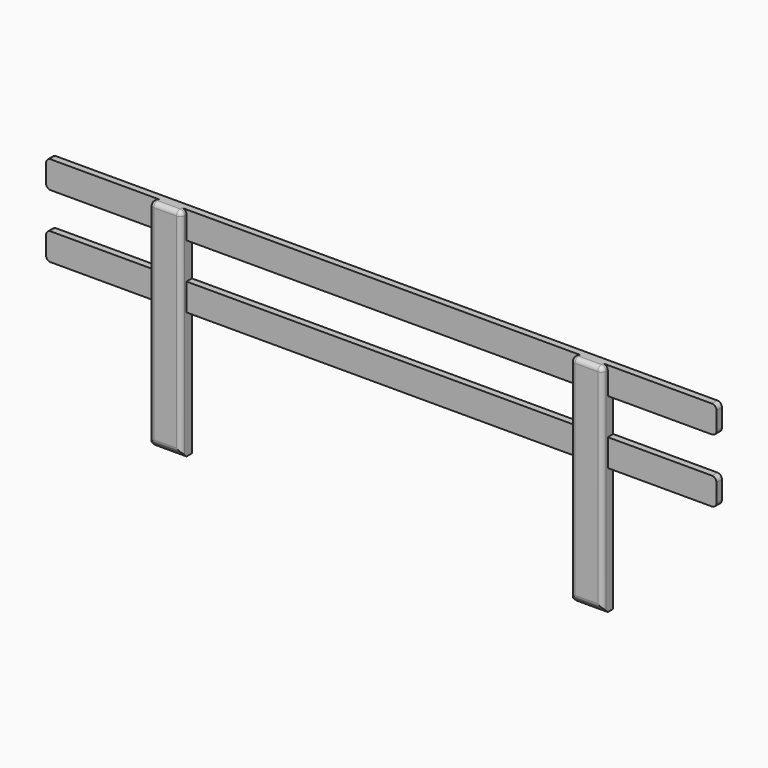
from build123d import *

# Parameters (mm, degrees)
F0_W     = 19.05
F0_H     = 76.2
F1_DEPTH = 939.8
F2_W     = 88.9
F2_H     = 38.1
F3_DEPTH = 609.6
F4_SIZE  = 19.05
F5_W     = 19.05
F5_H     = 76.2
F6_DEPTH = 939.8
F7_R     = 12.7


with BuildPart() as f1:
    # F0 (on Right) → F1 (new body, symmetric)
    with BuildSketch(Plane.YZ):
        with Locations((-9.525, 571.5)):
            Rectangle(F0_W, F0_H)
    extrude(amount=F1_DEPTH, both=True)

    # F2 (on face) → F3 (join, through all)
    with BuildSketch(Plane.XY.offset(609.6)):
        with Locations((590.55, -19.05)):
            Rectangle(F2_W, F2_H)
        with Locations((-590.55, -19.05)):
            Rectangle(F2_W, F2_H)
    extrude(amount=-F3_DEPTH)

    # F4
    f4_edges = [f1.edges().sort_by_distance(p)[0] for p in [
        (590.55, -38.1, 0),
        (-590.55, -38.1, 0),
    ]]
    chamfer(f4_edges, length=F4_SIZE)

    # F5 (on Right) → F6 (join, symmetric)
    with BuildSketch(Plane.YZ):
        with Locations((-9.525, 393.7)):
            Rectangle(F5_W, F5_H)
    extrude(amount=F6_DEPTH, both=True)

    # F7
    f7_edges = [f1.edges().sort_by_distance(p)[0] for p in [
        (939.8, -9.525, 609.6),
        (939.8, -9.525, 533.4),
        (590.55, -38.1, 609.6),
        (635, -28.575, 609.6),
        (546.1, -28.575, 609.6),
        (635, -38.1, 314.325),
        (546.1, -38.1, 314.325),
        (-590.55, -38.1, 609.6),
        (-546.1, -38.1, 314.325),
        (-635, -38.1, 314.325),
        (-635, -28.575, 609.6),
        (-939.8, -9.525, 609.6),
        (-939.8, -9.525, 533.4),
        (-546.1, -28.575, 609.6),
        (-590.55, -38.1, 19.05),
        (590.55, -38.1, 19.05),
        (939.8, -9.525, 431.8),
        (939.8, -9.525, 355.6),
        (-939.8, -9.525, 431.8),
        (-939.8, -9.525, 355.6),
    ]]
    fillet(f7_edges, radius=F7_R)


solid = f1.part
